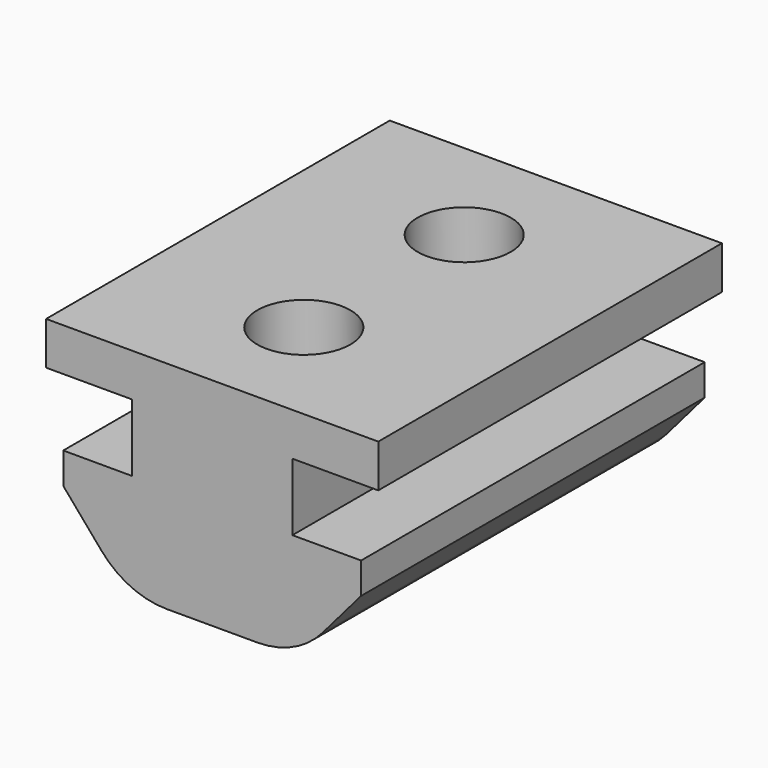
from build123d import *

# Parameters (mm, degrees)
F1_DEPTH = 15
F2_R     = 3
F3_R     = 1.625
F4_DEPTH = 6
F6_DEPTH = 3


# Not quite as in the source:
# - a feature names something its author has since deleted; it is built from what else it names


with BuildPart() as f1:
    # F0 (on Front) → F1 (new body)
    with BuildSketch(Plane.XZ):
        Polygon((2.8, 7.8979998849), (2.8, 10), (2.8, 10.25), (5.8, 10.25), (5.8, 11.75), (0, 11.75), (-5.8, 11.75), (-5.8, 10.25), (-2.8, 10.25), (-2.8, 10), (-2.8, 7.8979998849), (-5.2, 7.8997776918), (-5.2, 6.8109772229), (-2.9620195233, 4.2), (0, 4.2), (2.9620195233, 4.2), (5.2, 6.8109772229), (5.2, 7.8997776918), align=None)
    extrude(amount=F1_DEPTH)

    # F2
    f2_edges = [f1.edges().sort_by_distance(p)[0] for p in [
        (-2.96202, -7.5, 4.2),
        (2.96202, -7.5, 4.2),
    ]]
    fillet(f2_edges, radius=F2_R)

    # F3 (on face) → F4 (cut)
    with BuildSketch(Plane.XY.offset(11.75)):
        with Locations((0, -4)):
            Circle(F3_R)
        with Locations((0, -11)):
            Circle(F3_R)
    extrude(amount=-F4_DEPTH, mode=Mode.SUBTRACT)

    # F5 (on face) → F6 (cut)
    with BuildSketch(Plane(origin=(0, 0, 4.2), x_dir=(1, 0, 0), z_dir=(0, 0, -1))):
        Polygon((3, 12.7320508076), (1.5822147558, 13.5506094999), (1.5822147558, 8.4493905001), (3, 9.2679491924), align=None)
        Polygon((-1.5822147558, 8.4493905001), (-1.5822147558, 13.5506094999), (-3, 12.7320508076), (-3, 9.2679491924), align=None)
        Polygon((-1.5822147558, 1.4493905001), (-1.5822147558, 6.5506094999), (-3, 5.7320508076), (-3, 2.2679491924), align=None)
        Polygon((3, 5.7320508076), (1.5822147558, 6.5506094999), (1.5822147558, 1.4493905001), (3, 2.2679491924), align=None)
        Polygon((1.5822147558, 13.5506094999), (0, 14.4641016151), (-1.5822147558, 13.5506094999), (-1.5822147558, 8.4493905001), (0, 7.5358983849), (1.5822147558, 8.4493905001), align=None)
        Polygon((1.5822147558, 1.4493905001), (1.5822147558, 6.5506094999), (0, 7.4641016151), (-1.5822147558, 6.5506094999), (-1.5822147558, 1.4493905001), (0, 0.5358983849), align=None)
    extrude(amount=-F6_DEPTH, mode=Mode.SUBTRACT)


solid = f1.part
